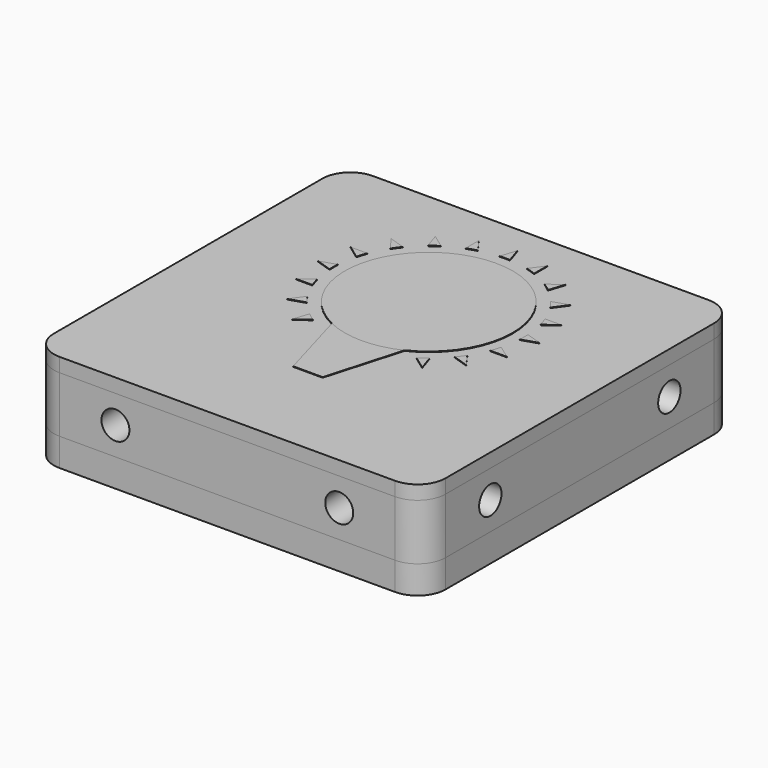
from build123d import *

# Parameters (mm, degrees)
F1_DEPTH  = 6.35
F2_W      = 6.35
F2_H      = 76.2
F3_DEPTH  = 12.7
F5_DEPTH  = 3.175
F6_R      = 3.175
F7_DEPTH  = 88.901
F8_R      = 3.175
F9_DEPTH  = 88.901
F10_W     = 18.2794369757
F10_H     = 12.4565269798
F10_H_2   = 11.1589711159
F10_H_3   = 10.510193184
F11_DEPTH = 1.27
F13_DEPTH = 3.175
F15_DEPTH = 1.27
F17_DEPTH = 1.397
F19_DEPTH = 1.397
F21_DEPTH = 0.127


with BuildPart() as f1:
    # F0 (on Top) → F1 (new body)
    with BuildSketch(Plane.XY):
        with BuildLine():
            Line((38.1, 44.45), (-38.1, 44.45))
            ThreePointArc((-38.1, 44.45), (-42.5901280605, 42.5901280605), (-44.45, 38.1))
            Line((-44.45, 38.1), (-44.45, -38.1))
            ThreePointArc((-44.45, -38.1), (-42.5901280605, -42.5901280605), (-38.1, -44.45))
            Line((-38.1, -44.45), (38.1, -44.45))
            ThreePointArc((38.1, -44.45), (42.5901280605, -42.5901280605), (44.45, -38.1))
            Line((44.45, -38.1), (44.45, 38.1))
            ThreePointArc((44.45, 38.1), (42.5901280605, 42.5901280605), (38.1, 44.45))
        make_face()
    extrude(amount=F1_DEPTH)


with BuildPart() as f3:
    # F2 (on face) → F3 (new body)
    with BuildSketch(Plane.XY.offset(6.35)):
        with BuildLine():
            Line((38.1, 44.45), (-38.1, 44.45))
            ThreePointArc((-38.1, 44.45), (-42.5901280605, 42.5901280605), (-44.45, 38.1))
            Line((-44.45, 38.1), (-38.1, 38.1))
            Line((-38.1, 38.1), (38.1, 38.1))
            Line((38.1, 38.1), (44.45, 38.1))
            ThreePointArc((44.45, 38.1), (42.5901280605, 42.5901280605), (38.1, 44.45))
        make_face()
        with Locations((-41.275, 0)):
            Rectangle(F2_W, F2_H)
        with BuildLine():
            Line((-38.1, -38.1), (-44.45, -38.1))
            ThreePointArc((-44.45, -38.1), (-42.5901280605, -42.5901280605), (-38.1, -44.45))
            Line((-38.1, -44.45), (38.1, -44.45))
            ThreePointArc((38.1, -44.45), (42.5901280605, -42.5901280605), (44.45, -38.1))
            Line((44.45, -38.1), (38.1, -38.1))
            Line((38.1, -38.1), (-38.1, -38.1))
        make_face()
        with Locations((41.275, 0)):
            Rectangle(F2_W, F2_H)
    extrude(amount=F3_DEPTH)

    # F6 (on face) → F7 (cut, through all)
    with BuildSketch(Plane.YZ.offset(44.45)):
        with Locations((25.4, 12.7)):
            Circle(F6_R)
        with Locations((-25.4, 12.7)):
            Circle(F6_R)
    extrude(amount=-F7_DEPTH, mode=Mode.SUBTRACT)

    # F8 (on face) → F9 (cut, through all)
    with BuildSketch(Plane(origin=(0, 44.45, 0), x_dir=(-1, 0, 0), z_dir=(0, 1, 0))):
        with Locations((25.4, 12.7)):
            Circle(F8_R)
        with Locations((-25.4, 12.7)):
            Circle(F8_R)
    extrude(amount=-F9_DEPTH, mode=Mode.SUBTRACT)


with BuildPart() as f5:
    # F4 (on face) → F5 (new body)
    with BuildSketch(Plane.XY.offset(19.05)):
        with BuildLine():
            Line((38.1, 44.45), (-38.1, 44.45))
            ThreePointArc((-38.1, 44.45), (-42.5901280605, 42.5901280605), (-44.45, 38.1))
            Line((-44.45, 38.1), (-44.45, -38.1))
            ThreePointArc((-44.45, -38.1), (-42.5901280605, -42.5901280605), (-38.1, -44.45))
            Line((-38.1, -44.45), (38.1, -44.45))
            ThreePointArc((38.1, -44.45), (42.5901280605, -42.5901280605), (44.45, -38.1))
            Line((44.45, -38.1), (44.45, 38.1))
            ThreePointArc((44.45, 38.1), (42.5901280605, 42.5901280605), (38.1, 44.45))
        make_face()
    extrude(amount=F5_DEPTH)

    # F10 (on face) → F11 (cut)
    with BuildSketch(Plane.XY.offset(22.225)):
        with BuildLine():
            Line((-3.81, 22.86), (-10.16, 22.86))
            ThreePointArc((-10.16, 22.86), (-11.9560512242, 22.1160512242), (-12.7, 20.32))
            Line((-12.7, 20.32), (-12.7, -20.32))
            ThreePointArc((-12.7, -20.32), (-11.9560512242, -22.1160512242), (-10.16, -22.86))
            Line((-10.16, -22.86), (10.16, -22.86))
            ThreePointArc((10.16, -22.86), (11.9560512242, -22.1160512242), (12.7, -20.32))
            Line((12.7, -20.32), (12.7, 20.32))
            ThreePointArc((12.7, 20.32), (11.9560512242, 22.1160512242), (10.16, 22.86))
            Line((10.16, 22.86), (3.81, 22.86))
            Line((3.81, 22.86), (3.81, 29.21))
            Line((3.81, 29.21), (-3.81, 29.21))
            Line((-3.81, 29.21), (-3.81, 22.86))
        make_face()
        Polygon((-2.3924338166, 21.5208735317), (-2.3924338166, 27.7491360903), (2.538274508, 27.7491360903), (2.538274508, 21.5208735317), (10.712868534, 21.5208735317), (10.712868534, -20.32), (-11.4753171802, -20.32), (-11.4753171802, 21.5208735317), align=None, mode=Mode.SUBTRACT)
        with Locations((0, 13.0867687985)):
            Rectangle(F10_W, F10_H)
        with Locations((0, -0.9268228896)):
            Rectangle(F10_W, F10_H_2)
        with Locations((0, -13.577981852)):
            Rectangle(F10_W, F10_H_3)
    extrude(amount=-F11_DEPTH, mode=Mode.SUBTRACT)


with BuildPart() as f13:
    # F12 (on face) → F13 (new body)
    with BuildSketch(Plane.XY.offset(19.05)):
        with BuildLine():
            Line((38.1, 44.45), (-38.1, 44.45))
            ThreePointArc((-38.1, 44.45), (-42.5901280605, 42.5901280605), (-44.45, 38.1))
            Line((-44.45, 38.1), (-44.45, -38.1))
            ThreePointArc((-44.45, -38.1), (-42.5901280605, -42.5901280605), (-38.1, -44.45))
            Line((-38.1, -44.45), (38.1, -44.45))
            ThreePointArc((38.1, -44.45), (42.5901280605, -42.5901280605), (44.45, -38.1))
            Line((44.45, -38.1), (44.45, 38.1))
            ThreePointArc((44.45, 38.1), (42.5901280605, 42.5901280605), (38.1, 44.45))
        make_face()
    extrude(amount=F13_DEPTH)

    # F14 (on face) → F15 (cut)
    with BuildSketch(Plane.XY.offset(22.225)):
        with BuildLine():
            ThreePointArc((8.255, -4.4685024099), (16.126999876, 2.5598631666), (19.05, 12.7))
            ThreePointArc((19.05, 12.7), (-10.1401368334, 28.826999876), (-8.255, -4.4685024099))
            ThreePointArc((-8.255, -4.4685024099), (-4.2333514554, -5.8736704896), (0, -6.35))
            ThreePointArc((0, -6.35), (4.2333514554, -5.8736704896), (8.255, -4.4685024099))
        make_face()
        with BuildLine():
            ThreePointArc((0, -6.35), (-4.2333514554, -5.8736704896), (-8.255, -4.4685024099))
            Line((-8.255, -4.4685024099), (-3.3454895688, -21.59))
            Line((-3.3454895688, -21.59), (0, -21.59))
            Line((0, -21.59), (0, -6.35))
        make_face()
        with BuildLine():
            Line((3.3454895688, -21.59), (8.255, -4.4685024099))
            ThreePointArc((8.255, -4.4685024099), (4.2333514554, -5.8736704896), (0, -6.35))
            Line((0, -6.35), (0, -21.59))
            Line((0, -21.59), (3.3454895688, -21.59))
        make_face()
    extrude(amount=-F15_DEPTH, mode=Mode.SUBTRACT)

    # F20 (on face) → F21 (join)
    with BuildSketch(Plane.XY.offset(22.225)):
        with BuildLine():
            ThreePointArc((-1.1698108915, 34.2809531223), (-0.5851199169, 34.3047131403), (0, 34.3126350821))
            Line((0, 34.3126350821), (0, 37.8738157451))
            Line((0, 37.8738157451), (-1.1698108915, 34.2809531223))
        make_face()
        with BuildLine():
            ThreePointArc((0, 34.3126350821), (0.5851199169, 34.3047131403), (1.1698108915, 34.2809531223))
            Line((1.1698108915, 34.2809531223), (0, 37.8738157451))
            Line((0, 37.8738157451), (0, 34.3126350821))
        make_face()
        with BuildLine():
            ThreePointArc((-7.7814375408, 32.8632146492), (-6.6786715336, 33.2548374291), (-5.5563249984, 33.5861975405))
            Line((-5.5563249984, 33.5861975405), (-7.7791368785, 36.6417215044))
            Line((-7.7791368785, 36.6417215044), (-7.7814375408, 32.8632146492))
        make_face()
        with BuildLine():
            ThreePointArc((-13.6313628671, 29.4717602408), (-12.7035881644, 30.1849890746), (-11.7385690843, 30.8469554208))
            Line((-11.7385690843, 30.8469554208), (-14.7967976389, 33.0660447511))
            Line((-14.7967976389, 33.0660447511), (-13.6313628671, 29.4717602408))
        make_face()
        with BuildLine():
            ThreePointArc((5.5563249984, 33.5861975405), (6.6786715336, 33.2548374291), (7.7814375408, 32.8632146492))
            Line((7.7814375408, 32.8632146492), (7.7791368785, 36.6417215044))
            Line((7.7791368785, 36.6417215044), (5.5563249984, 33.5861975405))
        make_face()
        with BuildLine():
            ThreePointArc((11.7385690843, 30.8469554208), (12.7035881644, 30.1849890746), (13.6313628671, 29.4717602408))
            Line((13.6313628671, 29.4717602408), (14.7967976389, 33.0660447511))
            Line((14.7967976389, 33.0660447511), (11.7385690843, 30.8469554208))
        make_face()
        with BuildLine():
            ThreePointArc((16.7717602408, 26.3313628671), (17.4849890746, 25.4035881644), (18.1469554208, 24.4385690843))
            Line((18.1469554208, 24.4385690843), (20.3660447511, 27.4967976389))
            Line((20.3660447511, 27.4967976389), (16.7717602408, 26.3313628671))
        make_face()
        with BuildLine():
            ThreePointArc((20.1632146492, 20.4814375408), (20.5548374291, 19.3786715336), (20.8861975405, 18.2563249984))
            Line((20.8861975405, 18.2563249984), (23.9417215044, 20.4791368785))
            Line((23.9417215044, 20.4791368785), (20.1632146492, 20.4814375408))
        make_face()
        with BuildLine():
            ThreePointArc((21.5809531223, 13.8698108915), (21.6047131403, 13.2851199169), (21.6126350821, 12.7))
            ThreePointArc((21.6126350821, 12.7), (21.6047131403, 12.1148800831), (21.5809531223, 11.5301891085))
            Line((21.5809531223, 11.5301891085), (25.1738157451, 12.7))
            Line((25.1738157451, 12.7), (21.5809531223, 13.8698108915))
        make_face()
        with BuildLine():
            Line((23.9417215044, 4.9208631215), (20.8861975405, 7.1436750016))
            ThreePointArc((20.8861975405, 7.1436750016), (20.5548374291, 6.0213284664), (20.1632146492, 4.9185624592))
            Line((20.1632146492, 4.9185624592), (23.9417215044, 4.9208631215))
        make_face()
        with BuildLine():
            Line((20.3660447511, -2.0967976389), (18.1469554208, 0.9614309157))
            ThreePointArc((18.1469554208, 0.9614309157), (17.4849890746, -0.0035881644), (16.7717602408, -0.9313628671))
            Line((16.7717602408, -0.9313628671), (20.3660447511, -2.0967976389))
        make_face()
        with BuildLine():
            Line((14.7967976389, -7.6660447511), (13.6313628671, -4.0717602408))
            ThreePointArc((13.6313628671, -4.0717602408), (12.7035881644, -4.7849890746), (11.7385690843, -5.4469554208))
            Line((11.7385690843, -5.4469554208), (14.7967976389, -7.6660447511))
        make_face()
        with BuildLine():
            Line((-14.7967976389, -7.6660447511), (-11.7385690843, -5.4469554208))
            ThreePointArc((-11.7385690843, -5.4469554208), (-12.7035881644, -4.7849890746), (-13.6313628671, -4.0717602408))
            Line((-13.6313628671, -4.0717602408), (-14.7967976389, -7.6660447511))
        make_face()
        with BuildLine():
            Line((-20.3660447511, -2.0967976389), (-16.7717602408, -0.9313628671))
            ThreePointArc((-16.7717602408, -0.9313628671), (-17.4849890746, -0.0035881644), (-18.1469554208, 0.9614309157))
            Line((-18.1469554208, 0.9614309157), (-20.3660447511, -2.0967976389))
        make_face()
        with BuildLine():
            Line((-23.9417215044, 4.9208631215), (-20.1632146492, 4.9185624592))
            ThreePointArc((-20.1632146492, 4.9185624592), (-20.5548374291, 6.0213284664), (-20.8861975405, 7.1436750016))
            Line((-20.8861975405, 7.1436750016), (-23.9417215044, 4.9208631215))
        make_face()
        with BuildLine():
            Line((-25.1738157451, 12.7), (-21.5809531223, 11.5301891085))
            ThreePointArc((-21.5809531223, 11.5301891085), (-21.6126350821, 12.7), (-21.5809531223, 13.8698108915))
            Line((-21.5809531223, 13.8698108915), (-25.1738157451, 12.7))
        make_face()
        with BuildLine():
            Line((-23.9417215044, 20.4791368785), (-20.8861975405, 18.2563249984))
            ThreePointArc((-20.8861975405, 18.2563249984), (-20.5548374291, 19.3786715336), (-20.1632146492, 20.4814375408))
            Line((-20.1632146492, 20.4814375408), (-23.9417215044, 20.4791368785))
        make_face()
        with BuildLine():
            ThreePointArc((-18.1469554208, 24.4385690843), (-17.4849890746, 25.4035881644), (-16.7717602408, 26.3313628671))
            Line((-16.7717602408, 26.3313628671), (-20.3660447511, 27.4967976389))
            Line((-20.3660447511, 27.4967976389), (-18.1469554208, 24.4385690843))
        make_face()
    extrude(amount=F21_DEPTH)


with BuildPart() as f17:
    # F16 (on face) → F17 (new body)
    with BuildSketch(Plane.XY.offset(20.955)):
        with BuildLine():
            ThreePointArc((-8.255, -4.4685024099), (0, -6.35), (8.255, -4.4685024099))
            ThreePointArc((8.255, -4.4685024099), (16.126999876, 2.5598631666), (19.05, 12.7))
            ThreePointArc((19.05, 12.7), (-10.1401368334, 28.826999876), (-8.255, -4.4685024099))
        make_face()
    extrude(amount=F17_DEPTH)


with BuildPart() as f19:
    # F18 (on face) → F19 (new body)
    with BuildSketch(Plane.XY.offset(20.955)):
        with BuildLine():
            Line((3.3454895688, -21.59), (8.255, -4.4685024099))
            ThreePointArc((8.255, -4.4685024099), (0, -6.35), (-8.255, -4.4685024099))
            Line((-8.255, -4.4685024099), (-3.3454895688, -21.59))
            Line((-3.3454895688, -21.59), (3.3454895688, -21.59))
        make_face()
    extrude(amount=F19_DEPTH)


solid = Compound([f1.part, f3.part, f5.part, f13.part, f17.part, f19.part])
